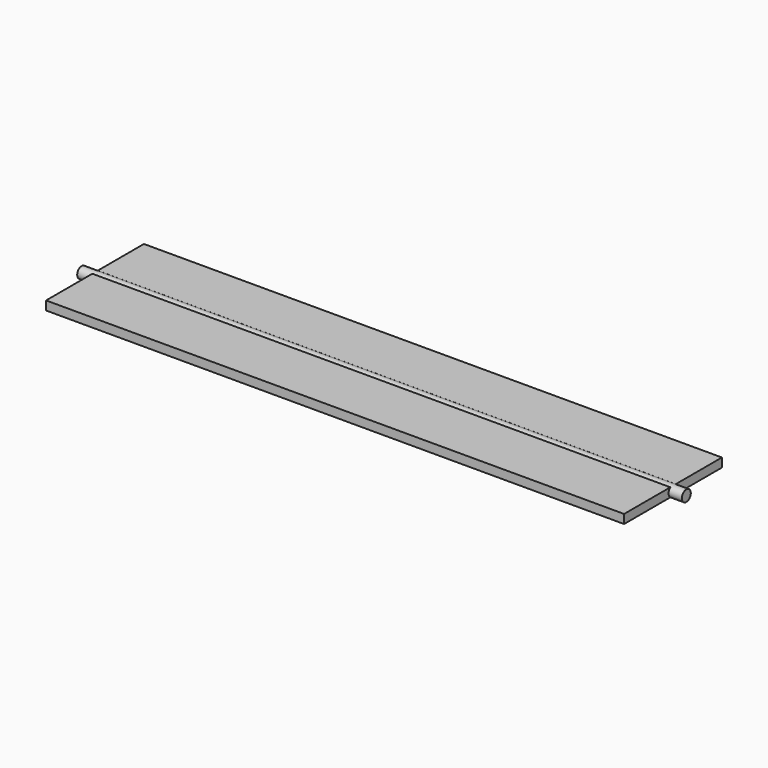
from build123d import *

# Parameters (mm, degrees)
F1_W     = 43.6626
F1_H     = 3.175
F2_DEPTH = 103.1875
F3_R     = 1.9812
F4_DEPTH = 107.95


# Not quite as in the source:
# - a variable given as a bare number and used for a length is read in inches; the dataset says mm whatever the document's units were


with BuildPart() as f2:
    # F1 (on Right) → F2 (new body, symmetric)
    with BuildSketch(Plane.YZ):
        Rectangle(F1_W, F1_H)
    extrude(amount=F2_DEPTH, both=True)

    # F3 (on Right) → F4 (join, symmetric)
    with BuildSketch(Plane.YZ):
        Circle(F3_R)
    extrude(amount=F4_DEPTH, both=True)


solid = f2.part
